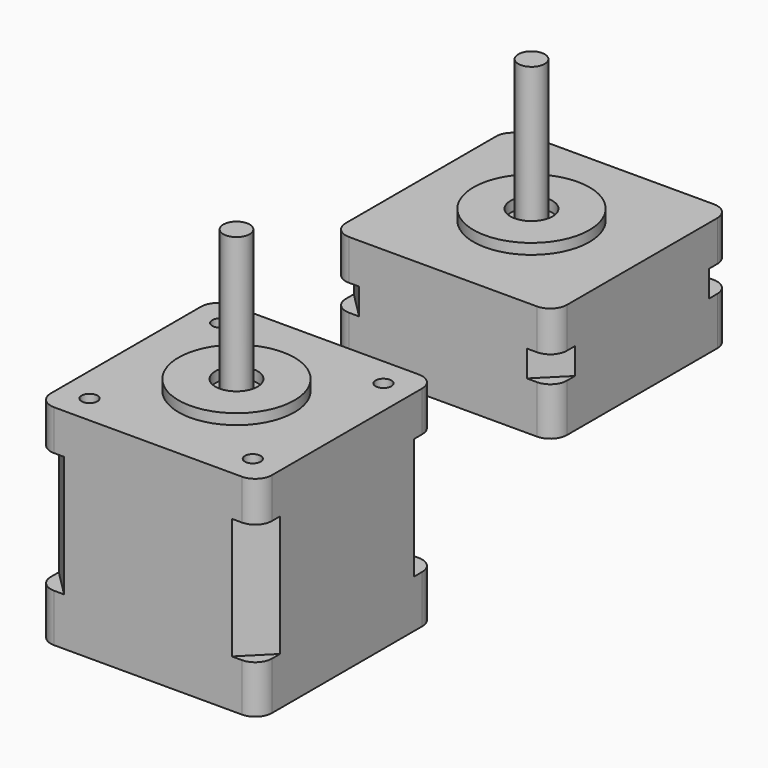
from build123d import *

# Parameters (mm, degrees)
F0_W      = 42
F0_H      = 42
F1_DEPTH  = 7.66
F2_R      = 11
F2_R_2    = 4
F3_DEPTH  = 2
F5_DEPTH  = 23
F6_DEPTH  = 5
F7_W      = 42
F7_H      = 42
F9_DEPTH  = 9.1
F8_W      = 42
F8_H      = 42
F10_R     = 3.175
F10_2_R   = 3.175
F11_D     = 3
F11_DEPTH = 10
F11_TIP   = 0.9012909285
F2_R_3    = 2.5
F12_DEPTH = 27


# Not quite as in the source:
# - a feature names something its author has since deleted; it is built from what else it names


with BuildPart() as f1:
    # F0 (on Top) → F1 (new body)
    with BuildSketch(Plane.XY):
        Rectangle(F0_W, F0_H)
    extrude(amount=F1_DEPTH)

    # F2 (on face) → F3 (join)
    with BuildSketch(Plane.XY.offset(7.66)):
        Circle(F2_R)
        Circle(F2_R_2, mode=Mode.SUBTRACT)
    extrude(amount=F3_DEPTH)

    # F4 (on face) → F5 (join)
    with BuildSketch(Plane(origin=(0, 0, 0), x_dir=(1, 0, 0), z_dir=(0, 0, -1))):
        Polygon((-21, -15.92), (-15.92, -21), (15.92, -21), (21, -15.92), (21, 15.92), (15.92, 21), (-15.92, 21), (-21, 15.92), align=None)
    extrude(amount=F5_DEPTH)

    # F7 (on face) → F9 (join)
    with BuildSketch(Plane(origin=(0, 0, -23), x_dir=(1, 0, 0), z_dir=(0, 0, -1))):
        Rectangle(F7_W, F7_H)
    extrude(amount=F9_DEPTH)

    # F10
    f10_edges = [f1.edges().sort_by_distance(p)[0] for p in [
        (21, 21, 3.83),
        (21, -21, 3.83),
        (-21, -21, 3.83),
        (-21, 21, 3.83),
        (21, -21, -27.55),
        (-21, 21, -27.55),
        (-21, -21, -27.55),
        (21, 21, -27.55),
    ]]
    fillet(f10_edges, radius=F10_R)

    # F11
    with Locations(Plane.XY.offset(7.66)):
        with Locations((15.5, 15.5), (-15.5, 15.5), (15.5, -15.5), (-15.5, -15.5), (15.5, 54.5), (-15.5, 54.5), (-15.5, 85.5), (15.5, 85.5)):
            Hole(F11_D / 2, depth=F11_DEPTH)
            with Locations((0, 0, -(F11_DEPTH + F11_TIP / 2))):  # 118° drill point
                Cone(0, F11_D / 2, F11_TIP, mode=Mode.SUBTRACT)

    # F2 (on face) → F12 (join)
    with BuildSketch(Plane.XY.offset(7.66)):
        Circle(F2_R_3)
    extrude(amount=F12_DEPTH)


with BuildPart() as f1b:
    # F0 (on Top) → F1, piece 2 (new body)
    with BuildSketch(Plane.XY):
        with Locations((0, 70)):
            Rectangle(F0_W, F0_H)
    extrude(amount=F1_DEPTH)

    # F2 (on face) → F3, piece 2 (join)
    with BuildSketch(Plane.XY.offset(7.66)):
        with Locations((0, 70)):
            Circle(F2_R)
        with Locations((0, 70)):
            Circle(F2_R_2, mode=Mode.SUBTRACT)
    extrude(amount=F3_DEPTH)

    # F4 (on face) → F6 (join)
    with BuildSketch(Plane(origin=(0, 0, 0), x_dir=(1, 0, 0), z_dir=(0, 0, -1))):
        Polygon((-21, -85.92), (-15.92, -91), (15.92, -91), (21, -85.92), (21, -54.08), (15.92, -49), (-15.92, -49), (-21, -54.08), align=None)
    extrude(amount=F6_DEPTH)

    # F8 (on face) → F9, piece 2 (join)
    with BuildSketch(Plane(origin=(0, 0, -5), x_dir=(1, 0, 0), z_dir=(0, 0, -1))):
        with Locations((0, -70)):
            Rectangle(F8_W, F8_H)
    extrude(amount=F9_DEPTH)

    # F10#2
    f10_2_edges = [f1b.edges().sort_by_distance(p)[0] for p in [
        (-21, 91, 3.83),
        (-21, 49, 3.83),
        (21, 91, 3.83),
        (21, 49, 3.83),
        (-21, 49, -9.55),
        (-21, 91, -9.55),
        (21, 91, -9.55),
        (21, 49, -9.55),
    ]]
    fillet(f10_2_edges, radius=F10_2_R)

    # F2 (on face) → F12, piece 2 (join)
    with BuildSketch(Plane.XY.offset(7.66)):
        with Locations((0, 70)):
            Circle(F2_R_3)
    extrude(amount=F12_DEPTH)


solid = Compound([f1.part, f1b.part])
